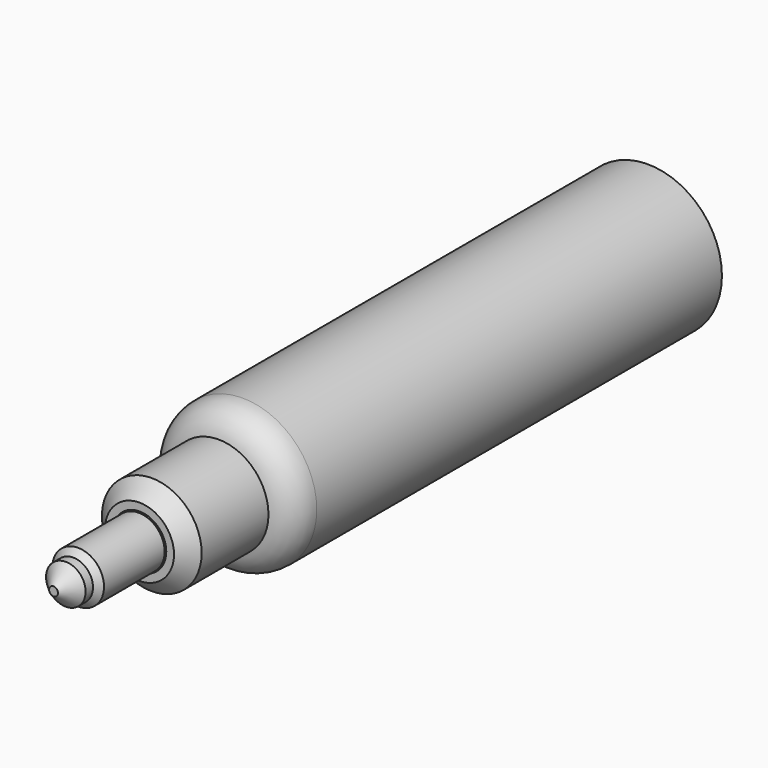
from build123d import *

# Parameters (mm, degrees)
F0_R         = 4.8298181264
F1_DEPTH     = 25
F2_DEPTH     = 10
F3_R         = 2
F4_R         = 1.5870534729
F5_DEPTH     = 0.5
F6_R         = 2.6450892659
F7_DEPTH     = 41.5
F8_R         = 1.6875975258
F9_DEPTH     = 47.4
F10_S7_R     = 1.6875975258
F10_T8_DEPTH = 5
F11_R        = 3.2484404645
F12_DEPTH    = 41.4
F13_SIZE     = 1
F14_R        = 1.2894560282
F15_DEPTH    = 48.4
F16_SIZE     = 1


# Not quite as in the source:
# - a fillet or chamfer that OpenCascade refuses, or shapes differently, is made with other operations: its cross-section is extruded or revolved along the edge and cut away or added


with BuildPart() as f1:
    # F0 (on Front) → F1 (new body)
    with BuildSketch(Plane.XZ):
        Circle(F0_R)
    extrude(amount=F1_DEPTH)

    # F2 (add): a face of the model
    f2_faces = [f1.faces().sort_by_distance(p)[0] for p in [
        (0, -25, 0),
    ]]
    extrude(f2_faces, amount=F2_DEPTH)

    # F3
    f3_edges = [f1.edges().sort_by_distance(p)[0] for p in [
        (-4.829818, -35, 0),
    ]]
    fillet(f3_edges, radius=F3_R)

    # F4 (on Front) → F5 (cut)
    with BuildSketch(Plane.XZ):
        Circle(F4_R)
    extrude(amount=F5_DEPTH, mode=Mode.SUBTRACT)

    # F6 (on Front) → F7 (join)
    with BuildSketch(Plane.XZ):
        Circle(F6_R)
    extrude(amount=F7_DEPTH)

    # F8 (on Front) → F9 (join)
    with BuildSketch(Plane.XZ):
        Circle(F8_R)
    extrude(amount=F9_DEPTH)

    # F10: chamfer of 1 on 2 edges, made by hand

    # F10_s1 → F10_t2 (revolve, cut)
    with BuildSketch(Plane.XY):
        Polygon((1.6875975258, -46.4), (0.6875975258, -47.4), (1.6875975258, -47.4), align=None)
    revolve(axis=Axis((0, -47.4, 0), (0, -1, 0)), mode=Mode.SUBTRACT)


with BuildPart() as f10_tool4:
    # F10_s5 → F10_t6 (revolve)
    with BuildSketch(Plane.XY):
        Polygon((2.6450892659, -40.5), (1.6450892659, -41.5), (2.6450892659, -41.5), align=None)
    revolve(axis=Axis((0, -41.5, 0), (0, -1, 0)))

    # F10_s7 → F10_t8 (cut, symmetric)
    with BuildSketch(Plane.XZ.offset(41)):
        Circle(F10_S7_R)
    extrude(amount=F10_T8_DEPTH, both=True, mode=Mode.SUBTRACT)


with BuildPart() as f1_1:
    add(f1.part)

    # F10_t3: cut F10_tool4
    add(f10_tool4.part, mode=Mode.SUBTRACT)

    # F11 (on Front) → F12 (join)
    with BuildSketch(Plane.XZ):
        Circle(F11_R)
    extrude(amount=F12_DEPTH)

    # F13
    f13_edges = [f1_1.edges().sort_by_distance(p)[0] for p in [
        (-3.24844, -41.4, 0),
    ]]
    chamfer(f13_edges, length=F13_SIZE)

    # F14 (on Front) → F15 (join)
    with BuildSketch(Plane.XZ):
        Circle(F14_R)
    extrude(amount=F15_DEPTH)

    # F16
    f16_edges = [f1_1.edges().sort_by_distance(p)[0] for p in [
        (-1.289456, -48.4, 0),
    ]]
    chamfer(f16_edges, length=F16_SIZE)


solid = f1_1.part
